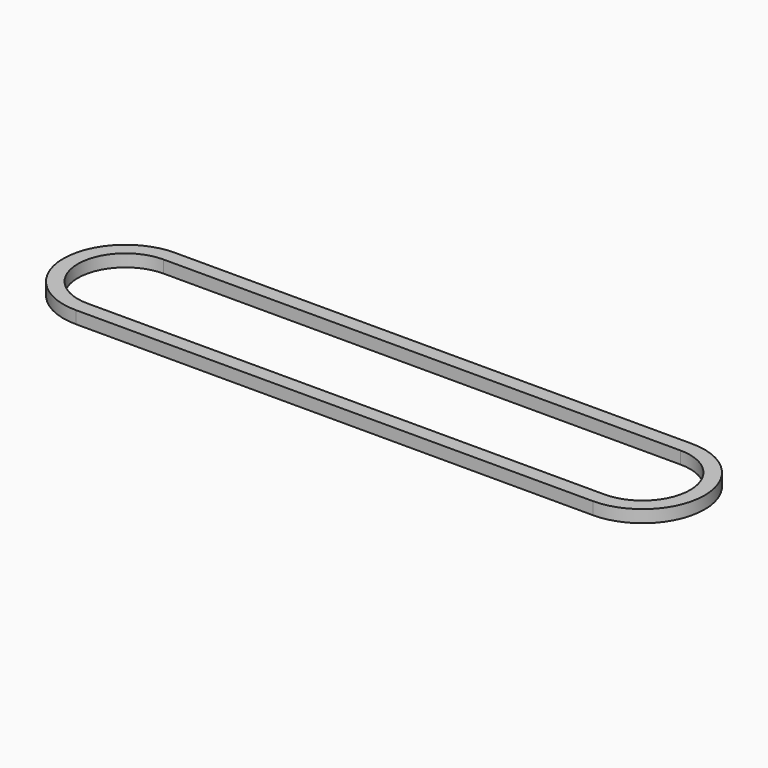
from build123d import *

# Parameters (mm, degrees)
F1_DEPTH = 60


# Not quite as in the source:
# - ends of sketch curves that miss each other by under 0.0002 mm in the source are joined


with BuildPart() as f1:
    # F0 (on Top) → F1 (new body)
    with BuildSketch(Plane.XY):
        with BuildLine():
            Line((2500, 299.9998967548), (0, 300))
            ThreePointArc((0, 300), (-300, 6.1947e-06), (0, -300))
            Line((0, -300), (2500.2488918055, -300))
            ThreePointArc((2500.2488918055, -300), (2800.2488659941, 0.1244459134), (2500, 299.9998967548))
        make_face()
        with BuildLine():
            ThreePointArc((0, -230), (-230, 4.7493e-06), (9.4986e-06, 230))
            Line((9.4986e-06, 230), (2500, 229.9998967548))
            ThreePointArc((2500, 229.9998967548), (2730.248889561, 0.1244459209), (2500.2488918055, -230.0000314225))
            Line((2500.2488918055, -230.0000314225), (2500.1035879766, -229.9999855242))
            Line((2500.1035879766, -229.9999855242), (0, -230))
        make_face(mode=Mode.SUBTRACT)
    extrude(amount=F1_DEPTH)


solid = f1.part
